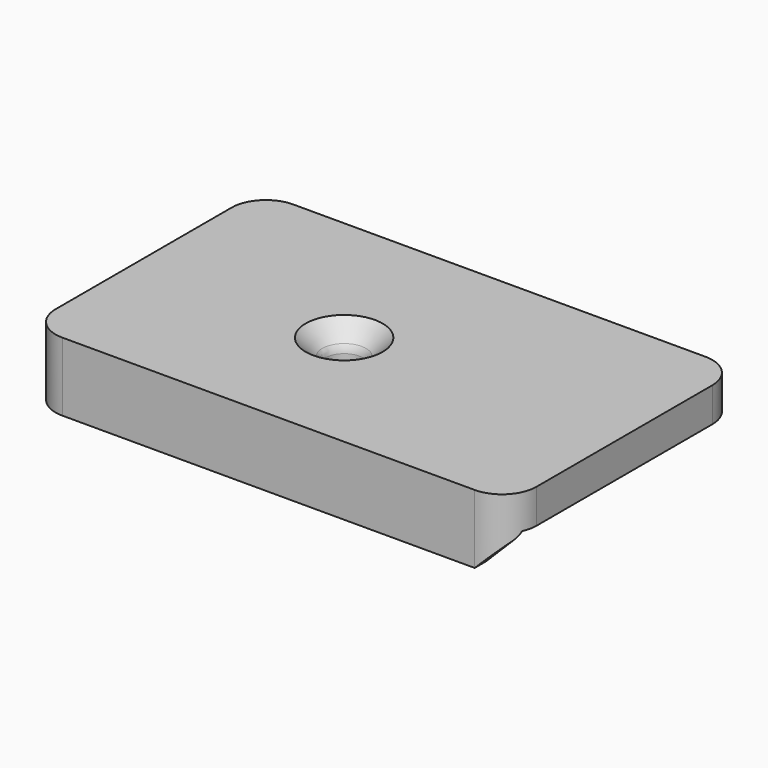
from build123d import *

# Parameters (mm, degrees)
F0_W           = 140
F0_H           = 84
F1_DEPTH       = 10
F2_D           = 11
F2_DEPTH       = 30
F2_CSINK_D     = 22.4
F2_CSINK_ANGLE = 90
F2_TIP         = 3.3047334047
F4_DEPTH       = 10
F5_SIZE        = 10
F6_T1_DEPTH    = 70
F6_T3_DEPTH    = 60
F7_R           = 3


# Not quite as in the source:
# - a fillet or chamfer that OpenCascade refuses, or shapes differently, is made with other operations: its cross-section is extruded or revolved along the edge and cut away or added


with BuildPart() as f1:
    # F0 (on Top) → F1 (new body)
    with BuildSketch(Plane.XY):
        with Locations((10, 2)):
            Rectangle(F0_W, F0_H)
    extrude(amount=-F1_DEPTH)

    # F2
    with Locations(Plane.XY):
        with Locations((0, 0)):
            CounterSinkHole(F2_D / 2, F2_CSINK_D / 2, depth=F2_DEPTH, counter_sink_angle=F2_CSINK_ANGLE)
            with Locations((0, 0, -(F2_DEPTH + F2_TIP / 2))):  # 118° drill point
                Cone(0, F2_D / 2, F2_TIP, mode=Mode.SUBTRACT)

    # F3 (on face) → F4 (join)
    with BuildSketch(Plane(origin=(0, 0, -10), x_dir=(1, 0, 0), z_dir=(0, 0, -1))):
        Polygon((80, 40), (-60, 40), (-60, -44), (-53, -44), (-53, 33), (80, 33), align=None)
    extrude(amount=F4_DEPTH)

    # F5
    f5_edges = [f1.edges().sort_by_distance(p)[0] for p in [
        (-56.5, 44, -20),
        (80, -36.5, -20),
    ]]
    chamfer(f5_edges, length=F5_SIZE)

    # F6: fillet of radius 10 on 4 edges, made by hand

    # F6_s2 → F6_t1 (cut)
    with BuildSketch(Plane.XY.offset(-45)):
        with BuildLine():
            ThreePointArc((-60, -30), (-57.0710678119, -37.0710678119), (-50, -40))
            Line((-50, -40), (-60, -40))
            Line((-60, -40), (-60, -30))
        make_face()
    extrude(amount=F6_T1_DEPTH, mode=Mode.SUBTRACT)

    # F6_s4 → F6_t3 (cut)
    with BuildSketch(Plane.XY.offset(-35)):
        with BuildLine():
            ThreePointArc((80, -30), (77.0710678119, -37.0710678119), (70, -40))
            Line((70, -40), (80, -40))
            Line((80, -40), (80, -30))
        make_face()
        with BuildLine():
            ThreePointArc((70, 44), (77.0710678119, 41.0710678119), (80, 34))
            Line((80, 34), (80, 44))
            Line((80, 44), (70, 44))
        make_face()
        with BuildLine():
            ThreePointArc((-50, 44), (-57.0710678119, 41.0710678119), (-60, 34))
            Line((-60, 34), (-60, 44))
            Line((-60, 44), (-50, 44))
        make_face()
    extrude(amount=F6_T3_DEPTH, mode=Mode.SUBTRACT)

    # F7
    f7_edges = [f1.edges().sort_by_distance(p)[0] for p in [
        (-53, -33, -15),
        (-53, 38.769696, -15.230304),
        (74.769696, -33, -15.230304),
        (-5.5, 0, -5.7),
    ]]
    fillet(f7_edges, radius=F7_R)


solid = f1.part
